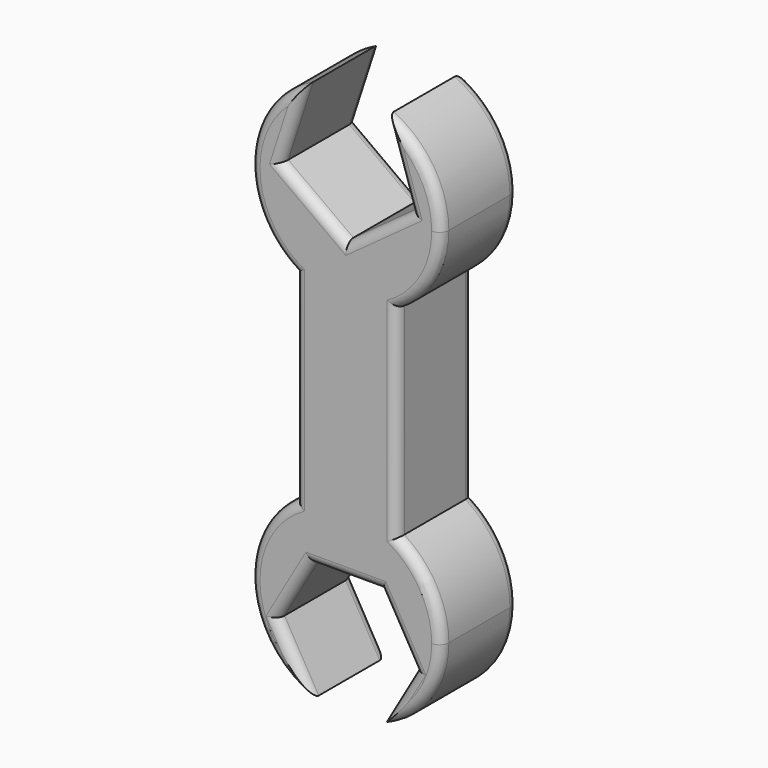
from build123d import *

# Parameters (mm, degrees)
F1_DEPTH = 25.4
F2_R     = 2.5399
F3_R     = 2.54


# Not quite as in the source:
# - a fillet or chamfer is up to 0.001 mm smaller than in the source, because OpenCascade refuses the exact size


with BuildPart() as f1:
    # F0 (on Front) → F1 (new body)
    with BuildSketch(Plane.XZ):
        with BuildLine():
            ThreePointArc((-13.5573409498, -17.4706149846), (0, -13.5498725689), (13.5573409498, -17.4706149846))
            Line((13.5573409498, -17.4706149846), (13.5573409498, 36.2410636034))
            ThreePointArc((13.5573409498, 36.2410636034), (0, 32.3203211877), (-13.5573409498, 36.2410636034))
            Line((-13.5573409498, 36.2410636034), (-13.5573409498, -17.4706149846))
        make_face()
        with BuildLine():
            ThreePointArc((-13.5573409498, 36.2410636034), (0, 32.3203211877), (13.5573409498, 36.2410636034))
            ThreePointArc((13.5573409498, 36.2410636034), (22.2431614224, 45.4564812533), (25.4, 57.7203211877))
            ThreePointArc((25.4, 57.7203211877), (21.419954319, 71.3711657393), (10.7271214983, 80.7439799838))
            Line((10.7271214983, 80.7439799838), (17.3568471858, 60.3397823797))
            Line((17.3568471858, 60.3397823797), (0, 47.7292947471))
            Line((0, 47.7292947471), (-17.3568471858, 60.3397823797))
            Line((-17.3568471858, 60.3397823797), (-10.7271214983, 80.7439799838))
            ThreePointArc((-10.7271214983, 80.7439799838), (-25.34879032, 59.3324096814), (-13.5573409498, 36.2410636034))
        make_face()
        with BuildLine():
            ThreePointArc((9.2408497758, -62.6092617289), (20.9747179278, -53.2754164625), (25.4, -38.9498725689))
            ThreePointArc((25.4, -38.9498725689), (22.2431614224, -26.6860326345), (13.5573409498, -17.4706149846))
            ThreePointArc((13.5573409498, -17.4706149846), (0, -13.5498725689), (-13.5573409498, -17.4706149846))
            ThreePointArc((-13.5573409498, -17.4706149846), (-25.2846540922, -41.3677781576), (-9.2408497758, -62.6092617289))
            Line((-9.2408497758, -62.6092617289), (-18.3499921745, -46.8317642808))
            Line((-18.3499921745, -46.8317642808), (-9.1749960873, -30.9402048984))
            Line((-9.1749960873, -30.9402048984), (9.1749960873, -30.9402048984))
            Line((9.1749960873, -30.9402048984), (18.3499921745, -46.8317642808))
            Line((18.3499921745, -46.8317642808), (9.2408497758, -62.6092617289))
        make_face()
    extrude(amount=F1_DEPTH)

    # F2 (radius 2.54 in the source; OpenCascade refuses exactly that, so slightly less here)
    f2_edges = [f1.edges().sort_by_distance(p)[0] for p in [
        (-13.762494, -25.4, -38.885985),
        (0, -25.4, -30.940205),
        (13.762494, -25.4, -38.885985),
        (-13.795421, -25.4, -54.720513),
        (13.795421, -25.4, -54.720513),
        (25.284654, -25.4, -41.367778),
        (-25.284654, -25.4, -41.367778),
        (-13.557341, -25.4, 9.385224),
        (-25.34879, -25.4, 59.33241),
        (-8.678424, -25.4, 54.034539),
        (-14.041984, -25.4, 70.541881),
        (14.041984, -25.4, 70.541881),
        (8.678424, -25.4, 54.034539),
        (25.34879, -25.4, 59.33241),
        (13.557341, -25.4, 9.385224),
    ]]
    fillet(f2_edges, radius=F2_R)

    # F3
    f3_edges = [f1.edges().sort_by_distance(p)[0] for p in [
        (25.34879, 0, 59.33241),
        (14.041984, 0, 70.541881),
        (8.678424, 0, 54.034539),
        (-14.041984, 0, 70.541881),
        (-8.678424, 0, 54.034539),
        (-25.34879, 0, 59.33241),
        (13.557341, 0, 9.385224),
        (-13.557341, 0, 9.385224),
        (25.284654, 0, -41.367778),
        (13.762494, 0, -38.885985),
        (13.795421, 0, -54.720513),
        (0, 0, -30.940205),
        (-13.762494, 0, -38.885985),
        (-25.284654, 0, -41.367778),
        (-13.795421, 0, -54.720513),
    ]]
    fillet(f3_edges, radius=F3_R)


solid = f1.part
